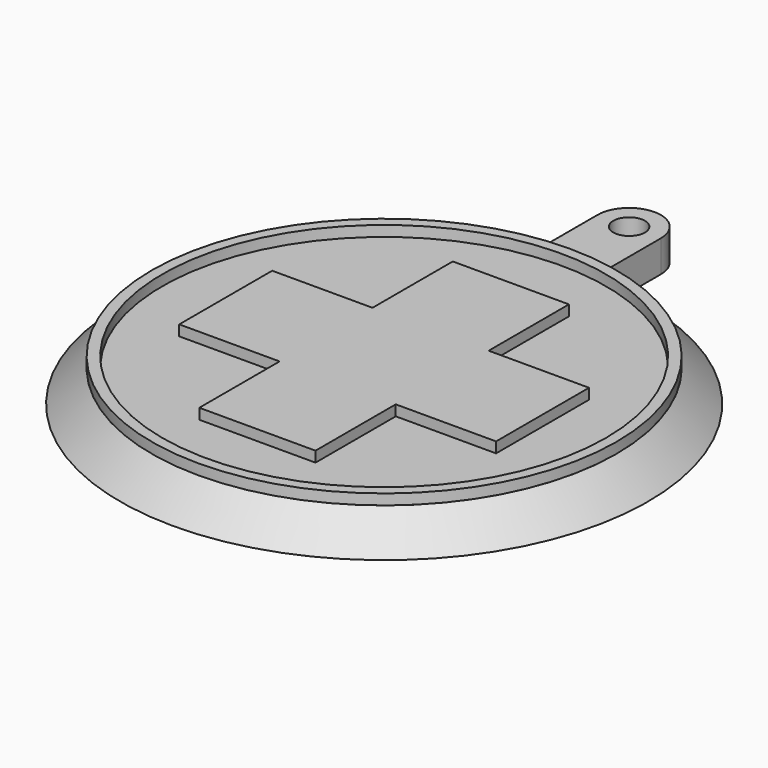
from build123d import *

# Parameters (mm, degrees)
F0_R     = 25
F1_DEPTH = 3
F2_W     = 11
F2_H     = 11
F2_H_2   = 9.5
F2_W_2   = 9.5
F3_DEPTH = 1
F2_R     = 22
F2_R_2   = 21
F4_R     = 1.5
F5_DEPTH = 3
F6_SIZE  = 2.99999


# Not quite as in the source:
# - a fillet or chamfer is up to 0.001 mm smaller than in the source, because OpenCascade refuses the exact size


with BuildPart() as f1:
    # F0 (on Top) → F1 (new body)
    with BuildSketch(Plane.XY):
        Circle(F0_R)
    extrude(amount=F1_DEPTH)

    # F4 (on Top) → F5 (join, through all)
    with BuildSketch(Plane.XY):
        with BuildLine():
            Line((3, 24.819347292), (3, 29))
            ThreePointArc((3, 29), (0, 26), (-3, 29))
            Line((-3, 29), (-3, 24.819347292))
            ThreePointArc((-3, 24.819347292), (0, 25), (3, 24.819347292))
        make_face()
        with BuildLine():
            ThreePointArc((-3, 29), (0, 26), (3, 29))
            ThreePointArc((3, 29), (0, 32), (-3, 29))
        make_face()
        with Locations((0, 29)):
            Circle(F4_R, mode=Mode.SUBTRACT)
    extrude(amount=F5_DEPTH)

    # F6 (size 3 in the source; OpenCascade refuses exactly that, so slightly less here)
    f6_edges = [f1.edges().sort_by_distance(p)[0] for p in [
        (0, -25, 3),
    ]]
    chamfer(f6_edges, length=F6_SIZE)


with BuildPart() as f3:
    # F2 (on face) → F3 (new body)
    with BuildSketch(Plane.XY.offset(3)):
        Rectangle(F2_W, F2_H)
        with Locations((0, 10.25)):
            Rectangle(F2_W, F2_H_2)
        with Locations((-10.25, 0)):
            Rectangle(F2_W_2, F2_H)
        with Locations((0, -10.25)):
            Rectangle(F2_W, F2_H_2)
        with Locations((10.25, 0)):
            Rectangle(F2_W_2, F2_H)
    extrude(amount=F3_DEPTH)


with BuildPart() as f3b:
    # F2 (on face) → F3, piece 2 (new body)
    with BuildSketch(Plane.XY.offset(3)):
        Circle(F2_R)
        Circle(F2_R_2, mode=Mode.SUBTRACT)
    extrude(amount=F3_DEPTH)


solid = Compound([f1.part, f3.part, f3b.part])
